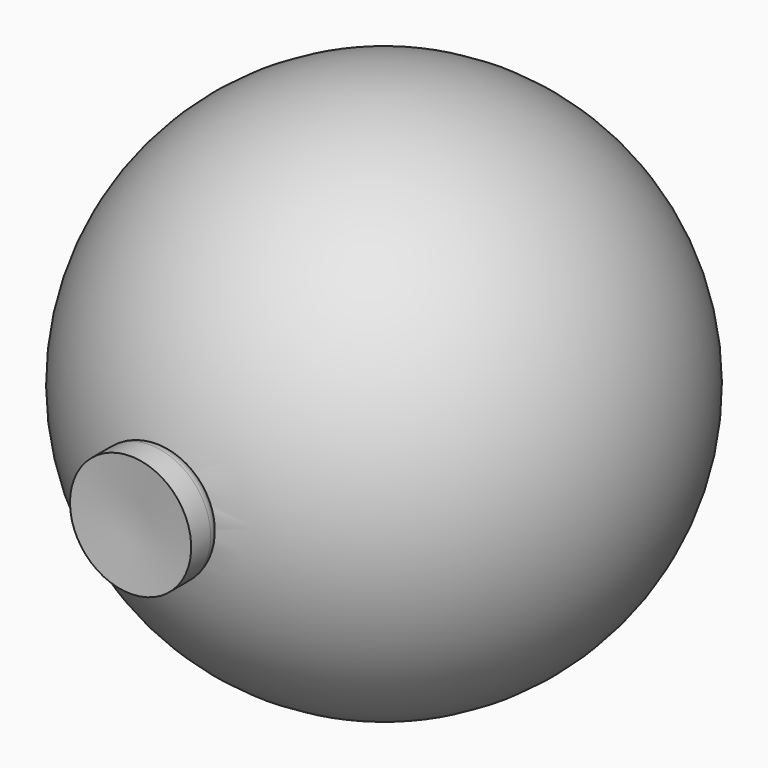
from build123d import *

# Parameters (mm, degrees)
F2_R     = 6.6860470745
F3_DEPTH = 59.436


# Not quite as in the source:
# - a feature of the source that left no trace in its solid (it failed there, or was rolled back) is left out


with BuildPart() as f1:
    # F0 (on Front) → F1 (revolve)
    with BuildSketch(Plane.XZ):
        with BuildLine():
            Line((0, -49.1313993841), (0, -47.4085077537))
            Line((0, -47.4085077537), (0, -42.4247202843))
            ThreePointArc((0, -42.4247202843), (-42.4247202843, 0), (0, 42.4247202843))
            Line((0, 42.4247202843), (0, 47.4085077537))
            Line((0, 47.4085077537), (0, 49.1313993841))
            ThreePointArc((0, 49.1313993841), (-49.1313993841, 0), (0, -49.1313993841))
        make_face()
    revolve(axis=Axis((0, 0, 44.916614019), (0, 0, -1)))

    # F2 (on Front) → F3 (cut, symmetric)
    with BuildSketch(Plane.XZ):
        Circle(F2_R)
    extrude(amount=F3_DEPTH, both=True, mode=Mode.SUBTRACT)

    # F5 (on Top) → F6 (revolve)
    with BuildSketch(Plane.XY):
        with BuildLine():
            ThreePointArc((-7.264834625, 49.0623677583), (-6.2348771191, 48.1257089546), (-5.8533530682, 46.7868357055))
            Line((-5.8533530682, 46.7868357055), (-5.8533530682, 0))
            Line((-5.8533530682, 0), (-5.8533530682, -31.4968999284))
            Line((-5.8533530682, -31.4968999284), (-6.1321007088, -48.0288676918))
            ThreePointArc((-6.1321007088, -48.0288676918), (-6.8938450816, -49.8000725931), (-8.6800149322, -50.5260330306))
            Line((-8.6800149322, -50.5260330306), (-9.7824803751, -50.5224412292))
            ThreePointArc((-9.7824803751, -50.5224412292), (-11.6117214108, -51.2916416407), (-12.3295195866, -53.1416572673))
            Line((-12.3295195866, -53.1416572673), (-12.3295195866, -57.6694607735))
            Line((-12.3295195866, -57.6694607735), (-1.0454875883, -56.8388439715))
            Line((-1.0454875883, -56.8388439715), (-1.0454875883, -34.0454652905))
            Line((-1.0454875883, -34.0454652905), (-1.0454875883, 53.5590164363))
            Line((-1.0454875883, 53.5590164363), (-11.8841901422, 53.5590164363))
            Line((-11.8841901422, 53.5590164363), (-11.8841901422, 52.9288002439))
            ThreePointArc((-11.8841901422, 52.9288002439), (-11.5026660913, 51.5899269948), (-10.4727085853, 50.653268191))
            Line((-10.4727085853, 50.653268191), (-7.264834625, 49.0623677583))
        make_face()
    revolve(axis=Axis((-1.0454875883, 9.7567755729, 0), (0, 1, 0)))


solid = f1.part
